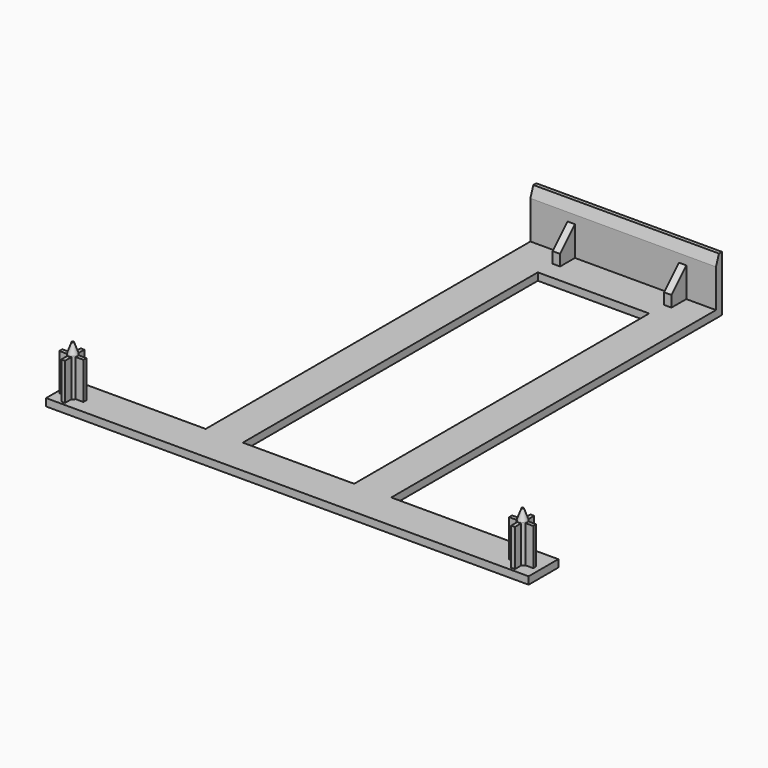
from build123d import *

# Parameters (mm, degrees)
F0_R       = 1.25
F1_DEPTH   = 2
F0_W       = 50
F0_H       = 2
F2_DEPTH   = 15
F3_SIZE2   = 2.7474774195
F3_SIZE    = 1
F3_2_SIZE2 = 2.7474774195
F3_2_SIZE  = 1
F3_3_SIZE2 = 2.7474774195
F3_3_SIZE  = 1
F4_W       = 2.75
F4_H       = 1
F4_W_2     = 1
F4_H_2     = 2.75
F5_DEPTH   = 10
F6_W       = 2
F6_H       = 5
F7_DEPTH   = 8
F8_SIZE    = 4.99999


# Not quite as in the source:
# - a fillet or chamfer is up to 0.001 mm smaller than in the source, because OpenCascade refuses the exact size
# - a feature names something its author has since deleted; it is built from what else it names


with BuildPart() as f1:
    # F0 (on Top) → F1 (new body)
    with BuildSketch(Plane.XY):
        Polygon((-30, 5), (-65, 5), (-65, -5), (65, -5), (65, 5), (20, 5), (10, 5), (-20, 5), align=None)
        with Locations((-61, -1)):
            Circle(F0_R, mode=Mode.SUBTRACT)
        with Locations((60.2, -1)):
            Circle(F0_R, mode=Mode.SUBTRACT)
        with Locations((-61, -1)):
            Circle(F0_R)
        with Locations((60.2, -1)):
            Circle(F0_R)
        Polygon((-30, 114.35), (-30, 5), (-20, 5), (-20, 104.35), (10, 104.35), (10, 5), (20, 5), (20, 114.35), align=None)
    extrude(amount=F1_DEPTH)

    # F0 (on Top) → F2 (join)
    with BuildSketch(Plane.XY):
        with Locations((60.2, -1)):
            Circle(F0_R)
        with Locations((-61, -1)):
            Circle(F0_R)
        with Locations((-5, 115.35)):
            Rectangle(F0_W, F0_H)
    extrude(amount=F2_DEPTH)

    # F3
    f3_edges = [f1.edges().sort_by_distance(p)[0] for p in [
        (58.95, -1, 15),
    ]]
    f3_side = f1.faces().sort_by_distance((60.2, -1, 15))[0]
    chamfer(f3_edges, length=F3_SIZE, length2=F3_SIZE2, reference=f3_side)

    # F3#2
    f3_2_edges = [f1.edges().sort_by_distance(p)[0] for p in [
        (-62.25, -1, 15),
    ]]
    f3_2_side = f1.faces().sort_by_distance((-61, -1, 15))[0]
    chamfer(f3_2_edges, length=F3_2_SIZE, length2=F3_2_SIZE2, reference=f3_2_side)

    # F3#3
    f3_3_edges = [f1.edges().sort_by_distance(p)[0] for p in [
        (-5, 114.35, 15),
    ]]
    f3_3_side = f1.faces().sort_by_distance((-5, 115.35, 15))[0]
    chamfer(f3_3_edges, length=F3_3_SIZE, length2=F3_3_SIZE2, reference=f3_3_side)

    # F4 (on face) → F5 (join)
    with BuildSketch(Plane.XY.offset(2)):
        with Locations((-62.875, -1)):
            Rectangle(F4_W, F4_H)
        with Locations((-61, 0.875)):
            Rectangle(F4_W_2, F4_H_2)
        with Locations((-61, -1)):
            Rectangle(F4_W_2, F4_H)
        with Locations((-59.125, -1)):
            Rectangle(F4_W, F4_H)
        with Locations((-61, -2.875)):
            Rectangle(F4_W_2, F4_H_2)
        with Locations((60.2, 0.875)):
            Rectangle(F4_W_2, F4_H_2)
        with Locations((60.2, -1)):
            Rectangle(F4_W_2, F4_H)
        with Locations((58.325, -1)):
            Rectangle(F4_W, F4_H)
        with Locations((62.075, -1)):
            Rectangle(F4_W, F4_H)
        with Locations((60.2, -2.875)):
            Rectangle(F4_W_2, F4_H_2)
    extrude(amount=F5_DEPTH)

    # F6 (on face) → F7 (join)
    with BuildSketch(Plane.XY.offset(2)):
        with Locations((-19, 111.85)):
            Rectangle(F6_W, F6_H)
        with Locations((11, 111.85)):
            Rectangle(F6_W, F6_H)
    extrude(amount=F7_DEPTH)

    # F8 (size 5 in the source; OpenCascade refuses exactly that, so slightly less here)
    f8_edges = [f1.edges().sort_by_distance(p)[0] for p in [
        (-19, 109.35, 10),
        (11, 109.35, 10),
    ]]
    chamfer(f8_edges, length=F8_SIZE)


solid = f1.part
